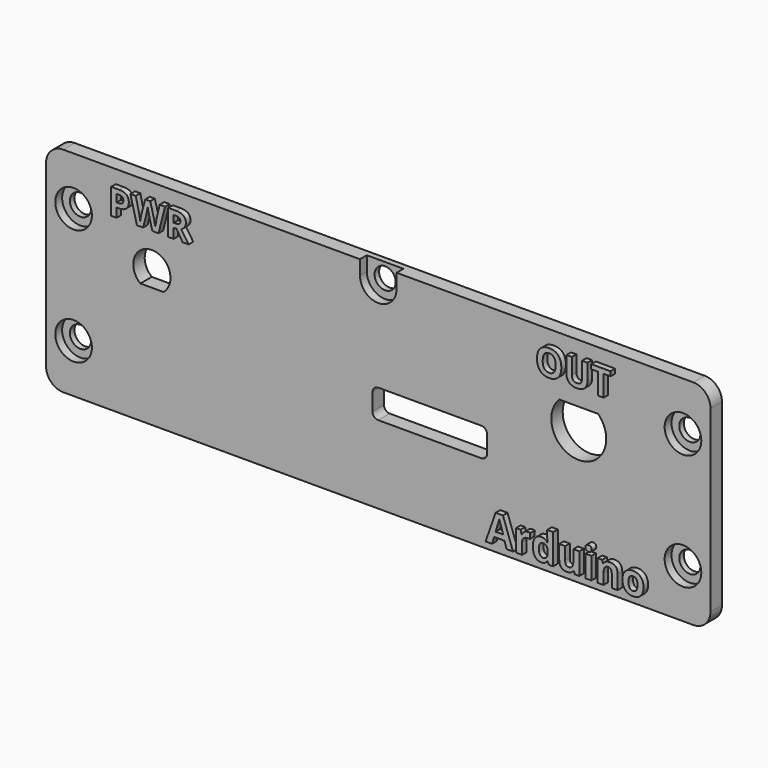
from build123d import *

# Parameters (mm, degrees)
F0_R          = 1.85
F1_DEPTH      = 2.5
F2_R          = 3.2
F3_DEPTH      = 1.5
F4_W          = 2.5
F4_H          = 6
F5_DEPTH      = 1.25
F7_DEPTH      = 2.501
F8_TEXT_SIZE  = 6.25
F9_DEPTH      = 1
F10_TEXT_SIZE = 6.9444444444
F11_DEPTH     = 1


# Not quite as in the source:
# - Text() gives the source's letters only with a copy of the font that has no kerning and outlines rounded to 1/6400 em; it was checked with that copy


with BuildPart() as f1:
    # F0 (on Front) → F1 (new body)
    with BuildSketch(Plane.XZ):
        with BuildLine():
            Line((55, 18.65), (-55, 18.65))
            ThreePointArc((-55, 18.65), (-57.1213203436, 17.7713203436), (-58, 15.65))
            Line((-58, 15.65), (-58, -15.65))
            ThreePointArc((-58, -15.65), (-57.1213203436, -17.7713203436), (-55, -18.65))
            Line((-55, -18.65), (55, -18.65))
            ThreePointArc((55, -18.65), (57.1213203436, -17.7713203436), (58, -15.65))
            Line((58, -15.65), (58, 15.65))
            ThreePointArc((58, 15.65), (57.1213203436, 17.7713203436), (55, 18.65))
        make_face()
        with Locations((-53.2, -10.15)):
            Circle(F0_R, mode=Mode.SUBTRACT)
        with Locations((53.2, -10.15)):
            Circle(F0_R, mode=Mode.SUBTRACT)
        with Locations((-53.2, 10.15)):
            Circle(F0_R, mode=Mode.SUBTRACT)
        with Locations((0, 16.15)):
            Circle(F0_R, mode=Mode.SUBTRACT)
        with Locations((53.2, 10.15)):
            Circle(F0_R, mode=Mode.SUBTRACT)
    extrude(amount=F1_DEPTH)

    # F2 (on face) → F3 (cut)
    with BuildSketch(Plane.XZ.offset(2.5)):
        with Locations((-53.2, 10.15)):
            Circle(F2_R)
        with Locations((53.2, 10.15)):
            Circle(F2_R)
        with Locations((-53.2, -10.15)):
            Circle(F2_R)
        with Locations((53.2, -10.15)):
            Circle(F2_R)
        with BuildLine():
            Line((-3.2, 18.65), (-3.2, 16.15))
            ThreePointArc((-3.2, 16.15), (0, 12.95), (3.2, 16.15))
            Line((3.2, 16.15), (3.2, 18.65))
            Line((3.2, 18.65), (-3.2, 18.65))
        make_face()
    extrude(amount=-F3_DEPTH, mode=Mode.SUBTRACT)

    # F4 (on face) → F5 (cut)
    with BuildSketch(Plane(origin=(0, 0, 0), x_dir=(-1, 0, 0), z_dir=(0, 1, 0))):
        with Locations((56.75, 0)):
            Rectangle(F4_W, F4_H)
    extrude(amount=-F5_DEPTH, mode=Mode.SUBTRACT)

    # F6 (on face) → F7 (cut, through all)
    with BuildSketch(Plane.XZ.offset(2.5)):
        with BuildLine():
            Line((-41.5450463315, 2.45), (-37.5151579956, 2.45))
            ThreePointArc((-37.5151579956, 2.45), (-39.5301021636, 8.25), (-41.5450463315, 2.45))
        make_face()
        with BuildLine():
            Line((38.3882148692, 8.4), (31.6117851308, 8.4))
            ThreePointArc((31.6117851308, 8.4), (35, 0.2), (38.3882148692, 8.4))
        make_face()
        with BuildLine():
            ThreePointArc((-1, -4.05), (-0.7071067812, -4.7571067812), (0, -5.05))
            Line((0, -5.05), (18, -5.05))
            ThreePointArc((18, -5.05), (18.7071067812, -4.7571067812), (19, -4.05))
            Line((19, -4.05), (19, -1.05))
            ThreePointArc((19, -1.05), (18.7071067812, -0.3428932188), (18, -0.05))
            Line((18, -0.05), (0, -0.05))
            ThreePointArc((0, -0.05), (-0.7071067812, -0.3428932188), (-1, -1.05))
            Line((-1, -1.05), (-1, -4.05))
        make_face()
    extrude(amount=-F7_DEPTH, mode=Mode.SUBTRACT)

    # F8 (on face) → F9 (join)
    with BuildSketch(Plane.XZ.offset(2.5)):
        with Locations((-46.4006096217, 11.8602635339)):
            Text('PWR', F8_TEXT_SIZE, font='Open Sans', font_style=FontStyle.BOLD, text_align=(TextAlign.LEFT, TextAlign.BOTTOM))
        with Locations((28.1498208642, 11.8602635339)):
            Text('OUT', F8_TEXT_SIZE, font='Open Sans', font_style=FontStyle.BOLD, text_align=(TextAlign.LEFT, TextAlign.BOTTOM))
    extrude(amount=F9_DEPTH)

    # F10 (on face) → F11 (join)
    with BuildSketch(Plane.XZ.offset(2.5)):
        with Locations((19.536309722, -16.9265348927)):
            Text('Arduino', F10_TEXT_SIZE, font='Open Sans', font_style=FontStyle.BOLD, text_align=(TextAlign.LEFT, TextAlign.BOTTOM))
    extrude(amount=F11_DEPTH)


solid = f1.part
